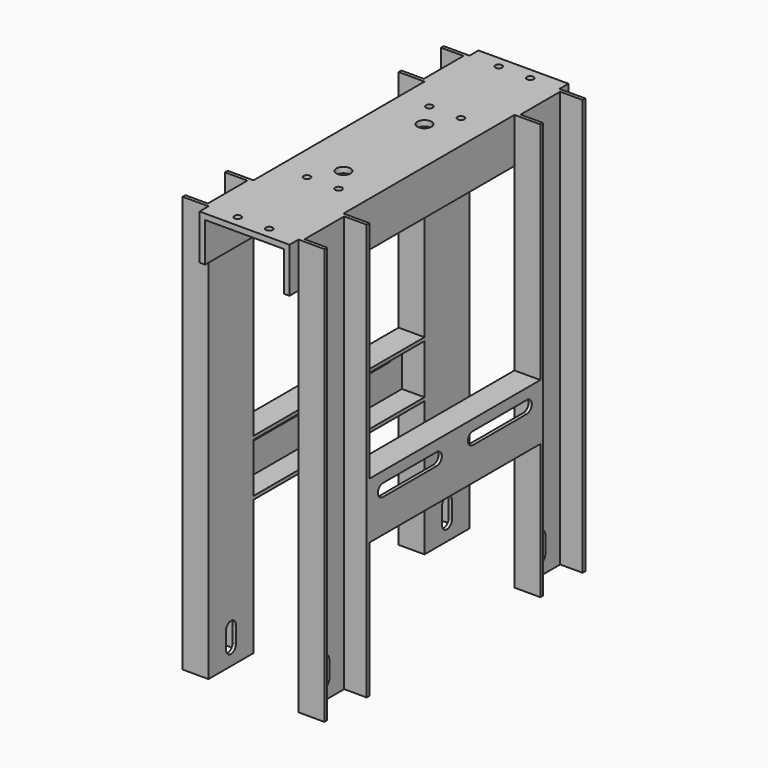
from build123d import *

# Parameters (mm, degrees)
F1_DEPTH  = 155
F3_DEPTH  = 370
F5_DEPTH  = 50
F6_R      = 6.25
F7_DEPTH  = 25
F8_R      = 3
F9_DEPTH  = 25
F11_DEPTH = 97.5
F13_DEPTH = 75


# Not quite as in the source:
# - a feature names something its author has since deleted; it is built from what else it names


with BuildPart() as f1:
    # F0 (on Front) → F1 (new body, symmetric)
    with BuildSketch(Plane.XZ):
        Polygon((40, -20), (40, 20), (-40, 20), (-40, -20), (-35, -20), (-35, 15), (35, 15), (35, -20), align=None)
    extrude(amount=F1_DEPTH, both=True)

    # F2 (on face) → F3 (join)
    with BuildSketch(Plane.XY.offset(20)):
        Polygon((-40, 145), (-63, 145), (-63, 142), (-43, 142), (-43, 97.9865193367), (-63, 97.9865193367), (-63, 95), (-43, 95), (-40, 95), align=None)
        Polygon((-40, -145), (-40, -95), (-43, -95), (-63, -95), (-63, -97.9865193367), (-43, -97.9865193367), (-43, -142), (-63, -142), (-63, -145), align=None)
        Polygon((43, -95), (40, -95), (40, -145), (63, -145), (63, -142), (43, -142), (43, -97.9865193367), (63, -97.9865193367), (63, -95), align=None)
        Polygon((63, 145), (40, 145), (40, 95), (43, 95), (63, 95), (63, 97.9865193367), (43, 97.9865193367), (43, 142), (63, 142), align=None)
    extrude(amount=-F3_DEPTH)

    # F4 (on Right) → F5 (cut, symmetric)
    with BuildSketch(Plane.YZ):
        with BuildLine():
            Line((114.5, -320), (114.5, -335))
            ThreePointArc((114.5, -335), (120, -340.5), (125.5, -335))
            Line((125.5, -335), (125.5, -320))
            ThreePointArc((125.5, -320), (120, -314.5), (114.5, -320))
        make_face()
        with BuildLine():
            Line((-114.5, -335), (-114.5, -320))
            ThreePointArc((-114.5, -320), (-120, -314.5), (-125.5, -320))
            Line((-125.5, -320), (-125.5, -335))
            ThreePointArc((-125.5, -335), (-120, -340.5), (-114.5, -335))
        make_face()
    extrude(amount=F5_DEPTH, both=True, mode=Mode.SUBTRACT)

    # F6 (on face) → F7 (cut)
    with BuildSketch(Plane.XY.offset(20)):
        with Locations((0, 45)):
            Circle(F6_R)
        with Locations((0, -45)):
            Circle(F6_R)
    extrude(amount=-F7_DEPTH, mode=Mode.SUBTRACT)

    # F8 (on face) → F9 (cut)
    with BuildSketch(Plane.XY.offset(20)):
        with Locations((-14, 145)):
            Circle(F8_R)
        with Locations((14, 145)):
            Circle(F8_R)
        with Locations((-14, 68)):
            Circle(F8_R)
        with Locations((14, 68)):
            Circle(F8_R)
        with Locations((-14, -68)):
            Circle(F8_R)
        with Locations((14, -68)):
            Circle(F8_R)
        with Locations((-14, -145)):
            Circle(F8_R)
        with Locations((14, -145)):
            Circle(F8_R)
    extrude(amount=-F9_DEPTH, mode=Mode.SUBTRACT)

    # F10 (on Front) → F11 (join, symmetric)
    with BuildSketch(Plane.XZ):
        Polygon((-40, -180), (-63, -180), (-63, -230), (-40, -230), (-40, -227), (-60, -227), (-60, -183), (-40, -183), align=None)
        Polygon((63, -180), (40, -180), (40, -183), (60, -183), (60, -227), (40, -227), (40, -230), (63, -230), align=None)
    extrude(amount=F11_DEPTH, both=True)

    # F12 (on Right) → F13 (cut, symmetric)
    with BuildSketch(Plane.YZ):
        with BuildLine():
            Line((19.9865193367, -200.5), (79.9865193367, -200.5))
            ThreePointArc((79.9865193367, -200.5), (85.4865193367, -195), (79.9865193367, -189.5))
            Line((79.9865193367, -189.5), (19.9865193367, -189.5))
            ThreePointArc((19.9865193367, -189.5), (14.4865193367, -195), (19.9865193367, -200.5))
        make_face()
        with BuildLine():
            ThreePointArc((-79.9865193367, -189.5), (-85.4865193367, -195), (-79.9865193367, -200.5))
            Line((-79.9865193367, -200.5), (-19.9865193367, -200.5))
            ThreePointArc((-19.9865193367, -200.5), (-14.4865193367, -195), (-19.9865193367, -189.5))
            Line((-19.9865193367, -189.5), (-79.9865193367, -189.5))
        make_face()
    extrude(amount=F13_DEPTH, both=True, mode=Mode.SUBTRACT)


solid = f1.part
